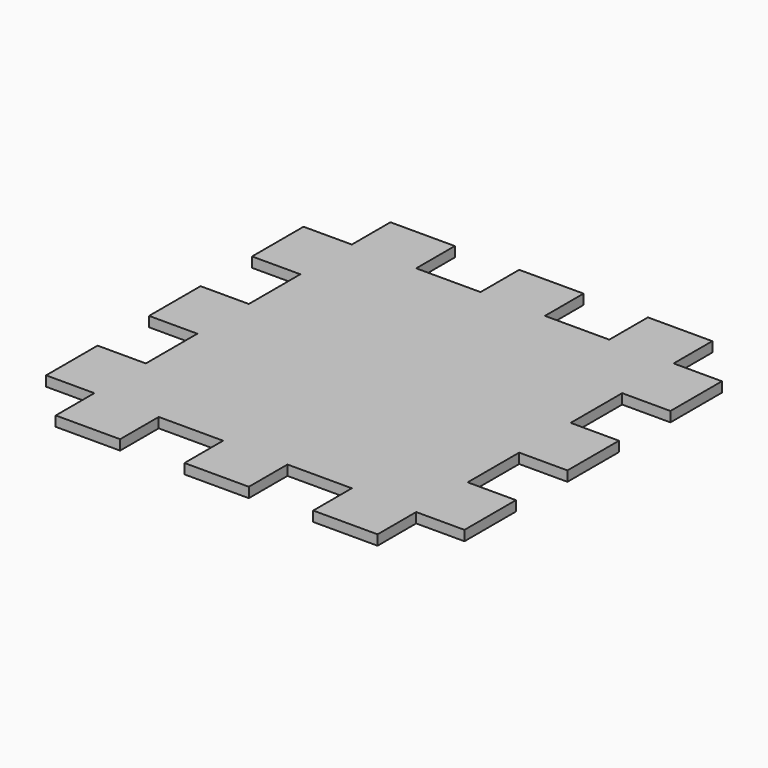
from build123d import *

# Parameters (mm, degrees)
F0_W     = 7.62
F0_H     = 10.16
F0_W_2   = 10.16
F0_H_2   = 7.62
F0_W_3   = 10.160000307
F0_W_4   = 7.619999693
F1_DEPTH = 1.5875


# Not quite as in the source:
# - ends of sketch curves that miss each other by under 0.0002 mm in the source are joined


with BuildPart() as f1:
    # F0 (on Top) → F1 (new body)
    with BuildSketch(Plane.XY):
        with Locations((29.21, -20.32)):
            Rectangle(F0_W, F0_H)
        with Locations((20.320000307, -29.21)):
            Rectangle(F0_W_2, F0_H_2)
        with Locations((3.07e-07, -29.21)):
            Rectangle(F0_W_2, F0_H_2)
        with Locations((-20.3199998465, -29.21)):
            Rectangle(F0_W_3, F0_H_2)
        with Locations((-29.2099998465, -20.32)):
            Rectangle(F0_W_4, F0_H)
        with Locations((-29.2099998465, 0)):
            Rectangle(F0_W_4, F0_H)
        with Locations((-29.2099998465, 20.32)):
            Rectangle(F0_W_4, F0_H)
        with Locations((-20.320000307, 29.21)):
            Rectangle(F0_W_2, F0_H_2)
        with Locations((-3.07e-07, 29.21)):
            Rectangle(F0_W_2, F0_H_2)
        with Locations((20.3199998465, 29.21)):
            Rectangle(F0_W_3, F0_H_2)
        with Locations((29.21, 20.32)):
            Rectangle(F0_W, F0_H)
        Polygon((25.4, 15.24), (25.4, 25.4), (15.239999693, 25.4), (5.079999693, 25.4), (-5.080000307, 25.4), (-15.240000307, 25.4), (-25.4, 25.4), (-25.4, 15.24), (-25.4, 5.08), (-25.4, -5.08), (-25.4, -15.24), (-25.4, -25.4), (-15.239999693, -25.4), (-5.079999693, -25.4), (5.080000307, -25.4), (15.240000307, -25.4), (25.4, -25.4), (25.4, -15.24), (25.4, -5.08), (25.4, 5.08), align=None)
        with Locations((29.21, 0)):
            Rectangle(F0_W, F0_H)
    extrude(amount=F1_DEPTH)


solid = f1.part
